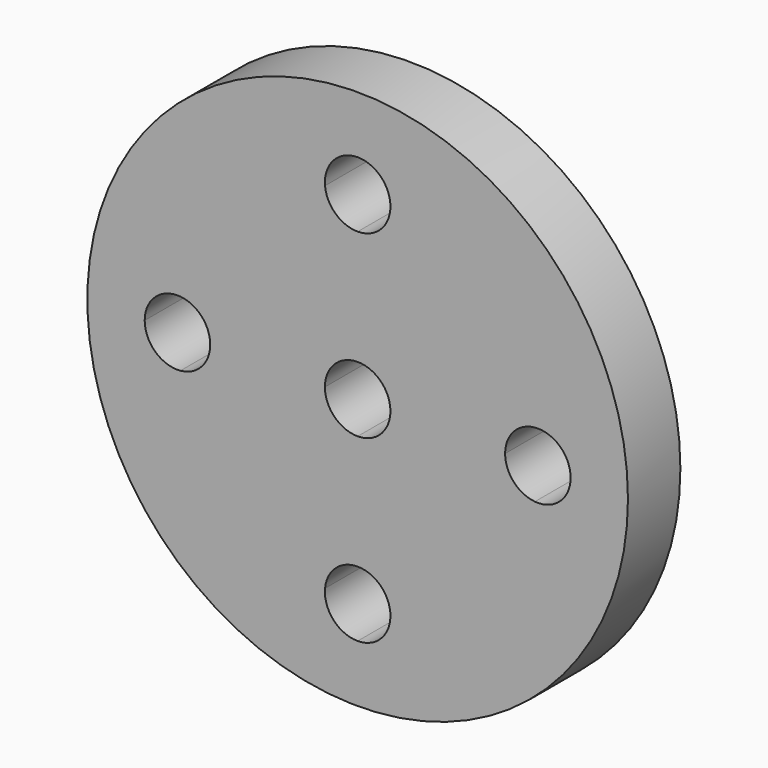
from build123d import *

# Parameters (mm, degrees)
F0_R     = 16.5
F1_DEPTH = 4
F3_DEPTH = 4.001


with BuildPart() as f1:
    # F0 (on Front) → F1 (new body)
    with BuildSketch(Plane.XZ):
        Circle(F0_R)
    extrude(amount=F1_DEPTH)

    # F2 (on face) → F3 (cut, through all)
    with BuildSketch(Plane.XZ.offset(4)):
        with BuildLine():
            ThreePointArc((-10.8181818182, -1.9917183909), (-9.5229021082, -1.3483997249), (-9, 0))
            Line((-9, 0), (-9.5, 0))
            Line((-9.5, 0), (-11, 0))
            ThreePointArc((-11, 0), (-10.9544511501, -1), (-10.8181818182, -1.9917183909))
        make_face()
        with BuildLine():
            Line((-9.5, 0), (-9, 0))
            ThreePointArc((-9, 0), (-9.5229021082, 1.3483997249), (-10.8181818182, 1.9917183909))
            ThreePointArc((-10.8181818182, 1.9917183909), (-10.9544511501, 1), (-11, 0))
            Line((-11, 0), (-9.5, 0))
        make_face()
        with BuildLine():
            ThreePointArc((0, 2), (-1.4142135624, 1.4142135624), (-2, 0))
            Line((-2, 0), (0, 0))
            Line((0, 0), (0, 2))
        make_face()
        with BuildLine():
            Line((0, 0), (-2, 0))
            ThreePointArc((-2, 0), (-1.4142135624, -1.4142135624), (0, -2))
            Line((0, -2), (0, 0))
        make_face()
        with BuildLine():
            ThreePointArc((-11, 0), (-10.9544511501, 1), (-10.8181818182, 1.9917183909))
            ThreePointArc((-10.8181818182, 1.9917183909), (-12.3483997249, 1.4770978918), (-13, 0))
            Line((-13, 0), (-11, 0))
        make_face()
        with BuildLine():
            ThreePointArc((-13, 0), (-12.3483997249, -1.4770978918), (-10.8181818182, -1.9917183909))
            ThreePointArc((-10.8181818182, -1.9917183909), (-10.9544511501, -1), (-11, 0))
            Line((-11, 0), (-13, 0))
        make_face()
        with BuildLine():
            Line((2, 0), (0, 0))
            Line((0, 0), (0, -2))
            ThreePointArc((0, -2), (1.4142135624, -1.4142135624), (2, 0))
        make_face()
        with BuildLine():
            Line((0, 2), (0, 0))
            Line((0, 0), (2, 0))
            ThreePointArc((2, 0), (1.4142135624, 1.4142135624), (0, 2))
        make_face()
        with BuildLine():
            ThreePointArc((0, 13), (-1.4770978918, 12.3483997249), (-1.9917183909, 10.8181818182))
            ThreePointArc((-1.9917183909, 10.8181818182), (-1, 10.9544511501), (0, 11))
            Line((0, 11), (0, 13))
        make_face()
        with BuildLine():
            ThreePointArc((0, 11), (-1, 10.9544511501), (-1.9917183909, 10.8181818182))
            ThreePointArc((-1.9917183909, 10.8181818182), (-1.3483997249, 9.5229021082), (0, 9))
            Line((0, 9), (0, 9.5))
            Line((0, 9.5), (0, 11))
        make_face()
        with BuildLine():
            ThreePointArc((0, -9), (-1.3483997249, -9.5229021082), (-1.9917183909, -10.8181818182))
            ThreePointArc((-1.9917183909, -10.8181818182), (-1, -10.9544511501), (0, -11))
            Line((0, -11), (0, -9.5))
            Line((0, -9.5), (0, -9))
        make_face()
        with BuildLine():
            ThreePointArc((0, -11), (-1, -10.9544511501), (-1.9917183909, -10.8181818182))
            ThreePointArc((-1.9917183909, -10.8181818182), (-1.4770978918, -12.3483997249), (0, -13))
            Line((0, -13), (0, -11))
        make_face()
        with BuildLine():
            Line((0, 9.5), (0, 9))
            ThreePointArc((0, 9), (1.3483997249, 9.5229021082), (1.9917183909, 10.8181818182))
            ThreePointArc((1.9917183909, 10.8181818182), (1, 10.9544511501), (0, 11))
            Line((0, 11), (0, 9.5))
        make_face()
        with BuildLine():
            ThreePointArc((1.9917183909, -10.8181818182), (1.3483997249, -9.5229021082), (0, -9))
            Line((0, -9), (0, -9.5))
            Line((0, -9.5), (0, -11))
            ThreePointArc((0, -11), (1, -10.9544511501), (1.9917183909, -10.8181818182))
        make_face()
        with BuildLine():
            Line((0, 13), (0, 11))
            ThreePointArc((0, 11), (1, 10.9544511501), (1.9917183909, 10.8181818182))
            ThreePointArc((1.9917183909, 10.8181818182), (1.997928525, 10.9089966535), (2, 11))
            ThreePointArc((2, 11), (1.4142135624, 12.4142135624), (0, 13))
        make_face()
        with BuildLine():
            ThreePointArc((1.9917183909, -10.8181818182), (1, -10.9544511501), (0, -11))
            Line((0, -11), (0, -13))
            ThreePointArc((0, -13), (1.4142135624, -12.4142135624), (2, -11))
            ThreePointArc((2, -11), (1.997928525, -10.9089966535), (1.9917183909, -10.8181818182))
        make_face()
        with BuildLine():
            ThreePointArc((10.8181818182, 1.9917183909), (9.5229021082, 1.3483997249), (9, 0))
            Line((9, 0), (9.5, 0))
            Line((9.5, 0), (11, 0))
            ThreePointArc((11, 0), (10.9544511501, 1), (10.8181818182, 1.9917183909))
        make_face()
        with BuildLine():
            Line((9.5, 0), (9, 0))
            ThreePointArc((9, 0), (9.5229021082, -1.3483997249), (10.8181818182, -1.9917183909))
            ThreePointArc((10.8181818182, -1.9917183909), (10.9544511501, -1), (11, 0))
            Line((11, 0), (9.5, 0))
        make_face()
        with BuildLine():
            ThreePointArc((13, 0), (12.3483997249, 1.4770978918), (10.8181818182, 1.9917183909))
            ThreePointArc((10.8181818182, 1.9917183909), (10.9544511501, 1), (11, 0))
            Line((11, 0), (13, 0))
        make_face()
        with BuildLine():
            ThreePointArc((11, 0), (10.9544511501, -1), (10.8181818182, -1.9917183909))
            ThreePointArc((10.8181818182, -1.9917183909), (12.3483997249, -1.4770978918), (13, 0))
            Line((13, 0), (11, 0))
        make_face()
    extrude(amount=-F3_DEPTH, mode=Mode.SUBTRACT)


solid = f1.part
